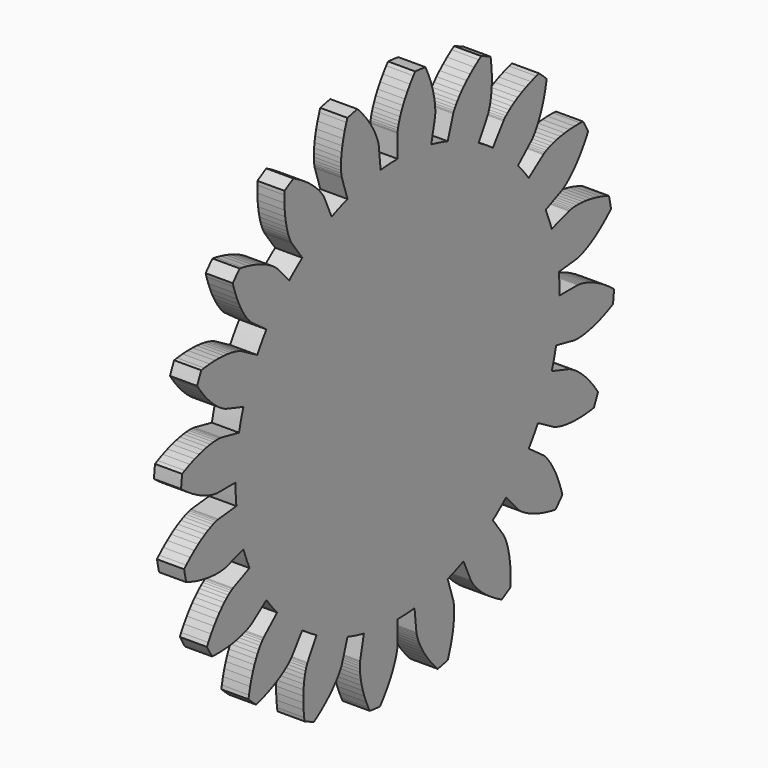
from build123d import *

# Parameters (mm, degrees)
F2_DEPTH = 12.7


# Not quite as in the source:
# - a variable given as a bare number and used for a length is read in inches; the dataset says mm whatever the document's units were


with BuildPart() as f2:
    # F1 (on Right) → F2 (new body)
    with BuildSketch(Plane.YZ):
        with BuildLine():
            ThreePointArc((92.7008893406, -19.704182302), (94.2527120653, -9.9063592233), (94.7718823529, 0))
            ThreePointArc((94.7718823529, 0), (94.6420007819, 4.9599770879), (94.2527120653, 9.9063592233))
            ThreePointArc((94.2527120653, 9.9063592233), (92.7008893406, 19.704182302), (90.1334162733, 29.286122236))
            ThreePointArc((90.1334162733, 29.286122236), (88.477174347, 33.9632051534), (86.5784226358, 38.5471972862))
            ThreePointArc((86.5784226358, 38.5471972862), (82.0748576821, 47.3859411765), (76.6720634124, 55.7055147791))
            ThreePointArc((76.6720634124, 55.7055147791), (73.6515856303, 59.6418780629), (70.4292339713, 63.4147671046))
            ThreePointArc((70.4292339713, 63.4147671046), (63.4147671046, 70.4292339713), (55.7055147791, 76.6720634124))
            ThreePointArc((55.7055147791, 76.6720634124), (51.6164665513, 79.4823883982), (47.3859411765, 82.0748576821))
            ThreePointArc((47.3859411765, 82.0748576821), (38.5471972862, 86.5784226358), (29.286122236, 90.1334162733))
            ThreePointArc((29.286122236, 90.1334162733), (24.5287680932, 91.5426087707), (19.704182302, 92.7008893406))
            ThreePointArc((19.704182302, 92.7008893406), (9.9063592233, 94.2527120653), (0, 94.7718823529))
            ThreePointArc((0, 94.7718823529), (-4.9599770879, 94.6420007819), (-9.9063592233, 94.2527120653))
            ThreePointArc((-9.9063592233, 94.2527120653), (-19.704182302, 92.7008893406), (-29.286122236, 90.1334162733))
            ThreePointArc((-29.286122236, 90.1334162733), (-33.9632051534, 88.477174347), (-38.5471972862, 86.5784226358))
            ThreePointArc((-38.5471972862, 86.5784226358), (-47.3859411765, 82.0748576821), (-55.7055147791, 76.6720634124))
            ThreePointArc((-55.7055147791, 76.6720634124), (-59.6418780629, 73.6515856303), (-63.4147671046, 70.4292339713))
            ThreePointArc((-63.4147671046, 70.4292339713), (-70.4292339713, 63.4147671046), (-76.6720634124, 55.7055147791))
            ThreePointArc((-76.6720634124, 55.7055147791), (-79.4823883982, 51.6164665513), (-82.0748576821, 47.3859411765))
            ThreePointArc((-82.0748576821, 47.3859411765), (-86.5784226358, 38.5471972862), (-90.1334162733, 29.286122236))
            ThreePointArc((-90.1334162733, 29.286122236), (-91.5426087707, 24.5287680932), (-92.7008893406, 19.704182302))
            ThreePointArc((-92.7008893406, 19.704182302), (-94.2527120653, 9.9063592233), (-94.7718823529, 0))
            ThreePointArc((-94.7718823529, 0), (-94.6420007819, -4.9599770879), (-94.2527120653, -9.9063592233))
            ThreePointArc((-94.2527120653, -9.9063592233), (-92.7008893406, -19.704182302), (-90.1334162733, -29.286122236))
            ThreePointArc((-90.1334162733, -29.286122236), (-88.477174347, -33.9632051534), (-86.5784226358, -38.5471972862))
            ThreePointArc((-86.5784226358, -38.5471972862), (-82.0748576821, -47.3859411765), (-76.6720634124, -55.7055147791))
            ThreePointArc((-76.6720634124, -55.7055147791), (-73.6515856303, -59.6418780629), (-70.4292339713, -63.4147671046))
            ThreePointArc((-70.4292339713, -63.4147671046), (-63.4147671046, -70.4292339713), (-55.7055147791, -76.6720634124))
            ThreePointArc((-55.7055147791, -76.6720634124), (-51.6164665513, -79.4823883982), (-47.3859411765, -82.0748576821))
            ThreePointArc((-47.3859411765, -82.0748576821), (-38.5471972862, -86.5784226358), (-29.286122236, -90.1334162733))
            ThreePointArc((-29.286122236, -90.1334162733), (-24.5287680932, -91.5426087707), (-19.704182302, -92.7008893406))
            ThreePointArc((-19.704182302, -92.7008893406), (-9.9063592233, -94.2527120653), (0, -94.7718823529))
            ThreePointArc((0, -94.7718823529), (4.9599770879, -94.6420007819), (9.9063592233, -94.2527120653))
            ThreePointArc((9.9063592233, -94.2527120653), (19.704182302, -92.7008893406), (29.286122236, -90.1334162733))
            ThreePointArc((29.286122236, -90.1334162733), (33.9632051534, -88.477174347), (38.5471972862, -86.5784226358))
            ThreePointArc((38.5471972862, -86.5784226358), (47.3859411765, -82.0748576821), (55.7055147791, -76.6720634124))
            ThreePointArc((55.7055147791, -76.6720634124), (59.6418780629, -73.6515856303), (63.4147671046, -70.4292339713))
            ThreePointArc((63.4147671046, -70.4292339713), (70.4292339713, -63.4147671046), (76.6720634124, -55.7055147791))
            ThreePointArc((76.6720634124, -55.7055147791), (79.4823883982, -51.6164665513), (82.0748576821, -47.3859411765))
            ThreePointArc((82.0748576821, -47.3859411765), (86.5784226358, -38.5471972862), (90.1334162733, -29.286122236))
            ThreePointArc((90.1334162733, -29.286122236), (91.5426087707, -24.5287680932), (92.7008893406, -19.704182302))
        make_face()
        with BuildLine():
            Line((-100.1470591498, -32.5397520376), (-90.1334162733, -29.286122236))
            ThreePointArc((-90.1334162733, -29.286122236), (-92.7008893406, -19.704182302), (-94.2527120653, -9.9063592233))
            Line((-94.2527120653, -9.9063592233), (-104.7240004928, -11.0069359858))
            Line((-104.7240004928, -11.0069359858), (-104.8543651896, -11.0250483896))
            Line((-104.8543651896, -11.0250483896), (-105.2426468777, -11.0967061046))
            Line((-105.2426468777, -11.0967061046), (-105.8831717727, -11.2476177493))
            Line((-105.8831717727, -11.2476177493), (-106.7683476445, -11.5030264298))
            Line((-106.7683476445, -11.5030264298), (-107.8886977686, -11.8875826074))
            Line((-107.8886977686, -11.8875826074), (-109.2329027705, -12.4252192764))
            Line((-109.2329027705, -12.4252192764), (-110.7878502107, -13.1390299218))
            Line((-110.7878502107, -13.1390299218), (-112.5386917362, -14.051149717))
            Line((-112.5386917362, -14.051149717), (-114.4689075917, -15.1826404116))
            Line((-114.4689075917, -15.1826404116), (-116.5603782638, -16.5533793458))
            Line((-116.5603782638, -16.5533793458), (-118.793463, -18.1819530161))
            Line((-118.793463, -18.1819530161), (-121.1470849264, -20.0855555985))
            Line((-121.1470849264, -20.0855555985), (-123.5988224587, -22.2798928209))
            Line((-123.5988224587, -22.2798928209), (-124.8108146855, -23.4789381691))
            ThreePointArc((-124.8108146855, -23.4789381691), (-124.2247452932, -26.4047847339), (-123.5700973145, -29.3160544701))
            Line((-123.5700973145, -29.3160544701), (-121.9751916412, -29.9184752517))
            Line((-121.9751916412, -29.9184752517), (-118.8429005996, -30.9258905601))
            Line((-118.8429005996, -30.9258905601), (-115.9184950556, -31.707613771))
            Line((-115.9184950556, -31.707613771), (-113.2160700507, -32.2871124607))
            Line((-113.2160700507, -32.2871124607), (-110.7478867658, -32.6886670274))
            Line((-110.7478867658, -32.6886670274), (-108.5243281119, -32.9372456942))
            Line((-108.5243281119, -32.9372456942), (-106.5538622456, -33.0583771854))
            Line((-106.5538622456, -33.0583771854), (-104.843014129, -33.0780215561))
            Line((-104.843014129, -33.0780215561), (-103.3963452215, -33.0224396629))
            Line((-103.3963452215, -33.0224396629), (-102.2164413659, -32.9180617635))
            Line((-102.2164413659, -32.9180617635), (-101.3039088997, -32.7913557409))
            Line((-101.3039088997, -32.7913557409), (-100.6573789956, -32.6686954428))
            Line((-100.6573789956, -32.6686954428), (-100.2735202047, -32.5762296325))
            Line((-100.2735202047, -32.5762296325), (-100.1470591498, -32.5397520376))
        make_face()
        with BuildLine():
            Line((-85.1901768198, -61.8942864279), (-76.6720634124, -55.7055147791))
            ThreePointArc((-76.6720634124, -55.7055147791), (-82.0748576821, -47.3859411765), (-86.5784226358, -38.5471972862))
            Line((-86.5784226358, -38.5471972862), (-96.1971128056, -42.8297140649))
            Line((-96.1971128056, -42.8297140649), (-96.3154999594, -42.8872248914))
            Line((-96.3154999594, -42.8872248914), (-96.6626343373, -43.0753610684))
            Line((-96.6626343373, -43.0753610684), (-97.2251754497, -43.4168196494))
            Line((-97.2251754497, -43.4168196494), (-97.9881021078, -43.9332621267))
            Line((-97.9881021078, -43.9332621267), (-98.9347839997, -44.6452040132))
            Line((-98.9347839997, -44.6452040132), (-100.0470600584, -45.5719090602))
            Line((-100.0470600584, -45.5719090602), (-101.3053233338, -46.7312885103))
            Line((-101.3053233338, -46.7312885103), (-102.6886120579, -48.139805771))
            Line((-102.6886120579, -48.139805771), (-104.1747065717, -49.8123868714))
            Line((-104.1747065717, -49.8123868714), (-105.7402317574, -51.7623370478))
            Line((-105.7402317574, -51.7623370478), (-107.3607646065, -54.0012637826))
            Line((-107.3607646065, -54.0012637826), (-109.010946528, -56.5390065966))
            Line((-109.010946528, -56.5390065966), (-110.6645999913, -59.3835738742))
            Line((-110.6645999913, -59.3835738742), (-111.4467477066, -60.898459961))
            ThreePointArc((-111.4467477066, -60.898459961), (-109.9852262806, -63.5), (-108.4629872309, -66.0664847026))
            Line((-108.4629872309, -66.0664847026), (-106.7599835382, -66.146567955))
            Line((-106.7599835382, -66.146567955), (-103.4696892814, -66.1367456855))
            Line((-103.4696892814, -66.1367456855), (-100.4468485755, -65.9765176277))
            Line((-100.4468485755, -65.9765176277), (-97.6976147214, -65.6925583801))
            Line((-97.6976147214, -65.6925583801), (-95.2261457396, -65.3117488872))
            Line((-95.2261457396, -65.3117488872), (-93.0346007599, -64.861043836))
            Line((-93.0346007599, -64.861043836), (-91.1231446684, -64.3673392905))
            Line((-91.1231446684, -64.3673392905), (-89.4899609743, -63.8573410545))
            Line((-89.4899609743, -63.8573410545), (-88.1312728324, -63.3574342551))
            Line((-88.1312728324, -63.3574342551), (-87.0413721267, -62.8935546306))
            Line((-87.0413721267, -62.8935546306), (-86.2126564928, -62.4910620021))
            Line((-86.2126564928, -62.4910620021), (-85.6356741311, -62.1746163987))
            Line((-85.6356741311, -62.1746163987), (-85.2991762334, -61.9680572974))
            Line((-85.2991762334, -61.9680572974), (-85.1901768198, -61.8942864279))
        make_face()
        with BuildLine():
            Line((-61.8942864279, -85.1901768198), (-55.7055147791, -76.6720634124))
            ThreePointArc((-55.7055147791, -76.6720634124), (-63.4147671046, -70.4292339713), (-70.4292339713, -63.4147671046))
            Line((-70.4292339713, -63.4147671046), (-78.2537814723, -70.4600213192))
            Line((-78.2537814723, -70.4600213192), (-78.3486025236, -70.5513010079))
            Line((-78.3486025236, -70.5513010079), (-78.6206096598, -70.8374995671))
            Line((-78.6206096598, -70.8374995671), (-79.050101546, -71.3360807394))
            Line((-79.050101546, -71.3360807394), (-79.6160984135, -72.0630040255))
            Line((-79.6160984135, -72.0630040255), (-80.2964442538, -73.0326417888))
            Line((-80.2964442538, -73.0326417888), (-81.0679140391, -74.257702867))
            Line((-81.0679140391, -74.257702867), (-81.9063255732, -75.7491629834))
            Line((-81.9063255732, -75.7491629834), (-82.7866555578, -77.5162022264))
            Line((-82.7866555578, -77.5162022264), (-83.6831594445, -79.5661498409))
            Line((-83.6831594445, -79.5661498409), (-84.5694946311, -81.9044365502))
            Line((-84.5694946311, -81.9044365502), (-85.4188465469, -84.5345546011))
            Line((-85.4188465469, -84.5345546011), (-86.2040571595, -87.4580256986))
            Line((-86.2040571595, -87.4580256986), (-86.8977554311, -90.6743769669))
            Line((-86.8977554311, -90.6743769669), (-87.1734965671, -92.3568161874))
            ThreePointArc((-87.1734965671, -92.3568161874), (-84.9795870076, -94.3793928356), (-82.738764251, -96.3498671001))
            Line((-82.738764251, -96.3498671001), (-81.0943644059, -95.8997737166))
            Line((-81.0943644059, -95.8997737166), (-77.9681438606, -94.8736753414))
            Line((-77.9681438606, -94.8736753414), (-75.1427647024, -93.7871802535))
            Line((-75.1427647024, -93.7871802535), (-72.6158361638, -92.6675589783))
            Line((-72.6158361638, -92.6675589783), (-70.3830060888, -91.5416617121))
            Line((-70.3830060888, -91.5416617121), (-68.4379984754, -90.4357910937))
            Line((-68.4379984754, -90.4357910937), (-66.7726587987, -89.3755777522))
            Line((-66.7726587987, -89.3755777522), (-65.3770069262, -88.3858590901))
            Line((-65.3770069262, -88.3858590901), (-64.2392974119, -87.4905617451))
            Line((-64.2392974119, -87.4905617451), (-63.3460869309, -86.7125881653))
            Line((-63.3460869309, -86.7125881653), (-62.6823085893, -86.0737077138))
            Line((-62.6823085893, -86.0737077138), (-62.2313528238, -85.5944527054))
            Line((-62.2313528238, -85.5944527054), (-61.9751545781, -85.2940197571))
            Line((-61.9751545781, -85.2940197571), (-61.8942864279, -85.1901768198))
        make_face()
        with BuildLine():
            Line((-32.5397520376, -100.1470591498), (-29.286122236, -90.1334162733))
            ThreePointArc((-29.286122236, -90.1334162733), (-38.5471972862, -86.5784226358), (-47.3859411765, -82.0748576821))
            Line((-47.3859411765, -82.0748576821), (-52.6504247823, -91.193210763))
            Line((-52.6504247823, -91.193210763), (-52.712397986, -91.309324222))
            Line((-52.712397986, -91.309324222), (-52.8826519268, -91.6655700544))
            Line((-52.8826519268, -91.6655700544), (-53.1370529285, -92.272469219))
            Line((-53.1370529285, -92.272469219), (-53.4507162886, -93.1387169979))
            Line((-53.4507162886, -93.1387169979), (-53.798129086, -94.2711357378))
            Line((-53.798129086, -94.2711357378), (-54.1532757602, -95.6746353334))
            Line((-54.1532757602, -95.6746353334), (-54.4897659907, -97.3521816082))
            Line((-54.4897659907, -97.3521816082), (-54.7809644032, -99.3047727207))
            Line((-54.7809644032, -99.3047727207), (-55.000121616, -101.531423694))
            Line((-55.000121616, -101.531423694), (-55.12050614, -104.0291591412))
            Line((-55.12050614, -104.0291591412), (-55.1155366392, -106.7930142284))
            Line((-55.1155366392, -106.7930142284), (-54.9589140573, -109.8160438893))
            Line((-54.9589140573, -109.8160438893), (-54.624753117, -113.0893402766))
            Line((-54.624753117, -113.0893402766), (-54.3670962101, -114.7746437576))
            ThreePointArc((-54.3670962101, -114.7746437576), (-51.6555536706, -116.0202731206), (-48.9154945515, -117.2018531969))
            Line((-48.9154945515, -117.2018531969), (-47.4906638679, -116.2656414539))
            Line((-47.4906638679, -116.2656414539), (-44.8345332828, -114.3237086311))
            Line((-44.8345332828, -114.3237086311), (-42.4831834698, -112.4173002224))
            Line((-42.4831834698, -112.4173002224), (-40.4259136183, -110.5716132508))
            Line((-40.4259136183, -110.5716132508), (-38.6502874148, -108.8108388804))
            Line((-38.6502874148, -108.8108388804), (-37.1422080646, -107.1580530158))
            Line((-37.1422080646, -107.1580530158), (-35.8859998534, -105.6351119473))
            Line((-35.8859998534, -105.6351119473), (-34.8644959317, -104.2625534176))
            Line((-34.8644959317, -104.2625534176), (-34.0591319791, -103.059503469))
            Line((-34.0591319791, -103.059503469), (-33.4500453881, -102.0435894082))
            Line((-33.4500453881, -102.0435894082), (-33.0161795879, -101.2308592037))
            Line((-33.0161795879, -101.2308592037), (-32.7353931107, -100.6357076096))
            Line((-32.7353931107, -100.6357076096), (-32.5845729864, -100.2708092847))
            Line((-32.5845729864, -100.2708092847), (-32.5397520376, -100.1470591498))
        make_face()
        with BuildLine():
            Line((0, -105.3008495645), (0, -94.7718823529))
            ThreePointArc((0, -94.7718823529), (-9.9063592233, -94.2527120653), (-19.704182302, -92.7008893406))
            Line((-19.704182302, -92.7008893406), (-21.8932776775, -102.9997733568))
            Line((-21.8932776775, -102.9997733568), (-21.9163366646, -103.1293545918))
            Line((-21.9163366646, -103.1293545918), (-21.9681717681, -103.5207758731))
            Line((-21.9681717681, -103.5207758731), (-22.0225793428, -104.1765855112))
            Line((-22.0225793428, -104.1765855112), (-22.0532056403, -105.0973634149))
            Line((-22.0532056403, -105.0973634149), (-22.0336782097, -106.2817140951))
            Line((-22.0336782097, -106.2817140951), (-21.9377375418, -107.7262678889))
            Line((-21.9377375418, -107.7262678889), (-21.7393684604, -109.4256904046))
            Line((-21.7393684604, -109.4256904046), (-21.4129307714, -111.3727001641))
            Line((-21.4129307714, -111.3727001641), (-20.9332886754, -113.558094385))
            Line((-20.9332886754, -113.558094385), (-20.2759384608, -115.9707828218))
            Line((-20.2759384608, -115.9707828218), (-19.4171339927, -118.5978295523))
            Line((-19.4171339927, -118.5978295523), (-18.3340095258, -121.4245025708))
            Line((-18.3340095258, -121.4245025708), (-17.0046993748, -124.4343310203))
            Line((-17.0046993748, -124.4343310203), (-16.2388656782, -125.9575295149))
            ThreePointArc((-16.2388656782, -125.9575295149), (-13.275114835, -126.3042807118), (-10.3040354309, -126.5813053094))
            Line((-10.3040354309, -126.5813053094), (-9.2382462636, -125.2506181353))
            Line((-9.2382462636, -125.2506181353), (-7.3122062067, -122.5829407799))
            Line((-7.3122062067, -122.5829407799), (-5.6650522415, -120.0432315881))
            Line((-5.6650522415, -120.0432315881), (-4.2788209839, -117.6521476207))
            Line((-4.2788209839, -117.6521476207), (-3.1342093163, -115.4288530094))
            Line((-3.1342093163, -115.4288530094), (-2.2106795434, -113.3909380948))
            Line((-2.2106795434, -113.3909380948), (-1.4865692099, -111.5543453819))
            Line((-1.4865692099, -111.5543453819), (-0.9392051602, -109.9333025766))
            Line((-0.9392051602, -109.9333025766), (-0.5450214043, -108.5402629356))
            Line((-0.5450214043, -108.5402629356), (-0.2796803426, -107.3858531403))
            Line((-0.2796803426, -107.3858531403), (-0.1181968911, -106.4788288778))
            Line((-0.1181968911, -106.4788288778), (-0.0350650391, -105.8260382829))
            Line((-0.0350650391, -105.8260382829), (-0.0043863607, -105.4323933716))
            Line((-0.0043863607, -105.4323933716), (0, -105.3008495645))
        make_face()
        with BuildLine():
            Line((32.5397520376, -100.1470591498), (29.286122236, -90.1334162733))
            ThreePointArc((29.286122236, -90.1334162733), (19.704182302, -92.7008893406), (9.9063592233, -94.2527120653))
            Line((9.9063592233, -94.2527120653), (11.0069359858, -104.7240004928))
            Line((11.0069359858, -104.7240004928), (11.0250483896, -104.8543651896))
            Line((11.0250483896, -104.8543651896), (11.0967061046, -105.2426468777))
            Line((11.0967061046, -105.2426468777), (11.2476177493, -105.8831717727))
            Line((11.2476177493, -105.8831717727), (11.5030264298, -106.7683476445))
            Line((11.5030264298, -106.7683476445), (11.8875826074, -107.8886977686))
            Line((11.8875826074, -107.8886977686), (12.4252192764, -109.2329027705))
            Line((12.4252192764, -109.2329027705), (13.1390299218, -110.7878502107))
            Line((13.1390299218, -110.7878502107), (14.051149717, -112.5386917362))
            Line((14.051149717, -112.5386917362), (15.1826404116, -114.4689075917))
            Line((15.1826404116, -114.4689075917), (16.5533793458, -116.5603782638))
            Line((16.5533793458, -116.5603782638), (18.1819530161, -118.793463))
            Line((18.1819530161, -118.793463), (20.0855555985, -121.1470849264))
            Line((20.0855555985, -121.1470849264), (22.2798928209, -123.5988224587))
            Line((22.2798928209, -123.5988224587), (23.4789381691, -124.8108146855))
            ThreePointArc((23.4789381691, -124.8108146855), (26.4047847339, -124.2247452932), (29.3160544701, -123.5700973145))
            Line((29.3160544701, -123.5700973145), (29.9184752517, -121.9751916412))
            Line((29.9184752517, -121.9751916412), (30.9258905601, -118.8429005996))
            Line((30.9258905601, -118.8429005996), (31.707613771, -115.9184950556))
            Line((31.707613771, -115.9184950556), (32.2871124607, -113.2160700507))
            Line((32.2871124607, -113.2160700507), (32.6886670274, -110.7478867658))
            Line((32.6886670274, -110.7478867658), (32.9372456942, -108.5243281119))
            Line((32.9372456942, -108.5243281119), (33.0583771854, -106.5538622456))
            Line((33.0583771854, -106.5538622456), (33.0780215561, -104.843014129))
            Line((33.0780215561, -104.843014129), (33.0224396629, -103.3963452215))
            Line((33.0224396629, -103.3963452215), (32.9180617635, -102.2164413659))
            Line((32.9180617635, -102.2164413659), (32.7913557409, -101.3039088997))
            Line((32.7913557409, -101.3039088997), (32.6686954428, -100.6573789956))
            Line((32.6686954428, -100.6573789956), (32.5762296325, -100.2735202047))
            Line((32.5762296325, -100.2735202047), (32.5397520376, -100.1470591498))
        make_face()
        with BuildLine():
            Line((61.8942864279, -85.1901768198), (55.7055147791, -76.6720634124))
            ThreePointArc((55.7055147791, -76.6720634124), (47.3859411765, -82.0748576821), (38.5471972862, -86.5784226358))
            Line((38.5471972862, -86.5784226358), (42.8297140649, -96.1971128056))
            Line((42.8297140649, -96.1971128056), (42.8872248914, -96.3154999594))
            Line((42.8872248914, -96.3154999594), (43.0753610684, -96.6626343373))
            Line((43.0753610684, -96.6626343373), (43.4168196494, -97.2251754497))
            Line((43.4168196494, -97.2251754497), (43.9332621267, -97.9881021078))
            Line((43.9332621267, -97.9881021078), (44.6452040132, -98.9347839997))
            Line((44.6452040132, -98.9347839997), (45.5719090602, -100.0470600584))
            Line((45.5719090602, -100.0470600584), (46.7312885103, -101.3053233338))
            Line((46.7312885103, -101.3053233338), (48.139805771, -102.6886120579))
            Line((48.139805771, -102.6886120579), (49.8123868714, -104.1747065717))
            Line((49.8123868714, -104.1747065717), (51.7623370478, -105.7402317574))
            Line((51.7623370478, -105.7402317574), (54.0012637826, -107.3607646065))
            Line((54.0012637826, -107.3607646065), (56.5390065966, -109.010946528))
            Line((56.5390065966, -109.010946528), (59.3835738742, -110.6645999913))
            Line((59.3835738742, -110.6645999913), (60.898459961, -111.4467477066))
            ThreePointArc((60.898459961, -111.4467477066), (63.5, -109.9852262806), (66.0664847026, -108.4629872309))
            Line((66.0664847026, -108.4629872309), (66.146567955, -106.7599835382))
            Line((66.146567955, -106.7599835382), (66.1367456855, -103.4696892814))
            Line((66.1367456855, -103.4696892814), (65.9765176277, -100.4468485755))
            Line((65.9765176277, -100.4468485755), (65.6925583801, -97.6976147214))
            Line((65.6925583801, -97.6976147214), (65.3117488872, -95.2261457396))
            Line((65.3117488872, -95.2261457396), (64.861043836, -93.0346007599))
            Line((64.861043836, -93.0346007599), (64.3673392905, -91.1231446684))
            Line((64.3673392905, -91.1231446684), (63.8573410545, -89.4899609743))
            Line((63.8573410545, -89.4899609743), (63.3574342551, -88.1312728324))
            Line((63.3574342551, -88.1312728324), (62.8935546306, -87.0413721267))
            Line((62.8935546306, -87.0413721267), (62.4910620021, -86.2126564928))
            Line((62.4910620021, -86.2126564928), (62.1746163987, -85.6356741311))
            Line((62.1746163987, -85.6356741311), (61.9680572974, -85.2991762334))
            Line((61.9680572974, -85.2991762334), (61.8942864279, -85.1901768198))
        make_face()
        with BuildLine():
            Line((85.1901768198, -61.8942864279), (76.6720634124, -55.7055147791))
            ThreePointArc((76.6720634124, -55.7055147791), (70.4292339713, -63.4147671046), (63.4147671046, -70.4292339713))
            Line((63.4147671046, -70.4292339713), (70.4600213192, -78.2537814723))
            Line((70.4600213192, -78.2537814723), (70.5513010079, -78.3486025236))
            Line((70.5513010079, -78.3486025236), (70.8374995671, -78.6206096598))
            Line((70.8374995671, -78.6206096598), (71.3360807394, -79.050101546))
            Line((71.3360807394, -79.050101546), (72.0630040255, -79.6160984135))
            Line((72.0630040255, -79.6160984135), (73.0326417888, -80.2964442538))
            Line((73.0326417888, -80.2964442538), (74.257702867, -81.0679140391))
            Line((74.257702867, -81.0679140391), (75.7491629834, -81.9063255732))
            Line((75.7491629834, -81.9063255732), (77.5162022264, -82.7866555578))
            Line((77.5162022264, -82.7866555578), (79.5661498409, -83.6831594445))
            Line((79.5661498409, -83.6831594445), (81.9044365502, -84.5694946311))
            Line((81.9044365502, -84.5694946311), (84.5345546011, -85.4188465469))
            Line((84.5345546011, -85.4188465469), (87.4580256986, -86.2040571595))
            Line((87.4580256986, -86.2040571595), (90.6743769669, -86.8977554311))
            Line((90.6743769669, -86.8977554311), (92.3568161874, -87.1734965671))
            ThreePointArc((92.3568161874, -87.1734965671), (94.3793928356, -84.9795870076), (96.3498671001, -82.738764251))
            Line((96.3498671001, -82.738764251), (95.8997737166, -81.0943644059))
            Line((95.8997737166, -81.0943644059), (94.8736753414, -77.9681438606))
            Line((94.8736753414, -77.9681438606), (93.7871802535, -75.1427647024))
            Line((93.7871802535, -75.1427647024), (92.6675589783, -72.6158361638))
            Line((92.6675589783, -72.6158361638), (91.5416617121, -70.3830060888))
            Line((91.5416617121, -70.3830060888), (90.4357910937, -68.4379984754))
            Line((90.4357910937, -68.4379984754), (89.3755777522, -66.7726587987))
            Line((89.3755777522, -66.7726587987), (88.3858590901, -65.3770069262))
            Line((88.3858590901, -65.3770069262), (87.4905617451, -64.2392974119))
            Line((87.4905617451, -64.2392974119), (86.7125881653, -63.3460869309))
            Line((86.7125881653, -63.3460869309), (86.0737077138, -62.6823085893))
            Line((86.0737077138, -62.6823085893), (85.5944527054, -62.2313528238))
            Line((85.5944527054, -62.2313528238), (85.2940197571, -61.9751545781))
            Line((85.2940197571, -61.9751545781), (85.1901768198, -61.8942864279))
        make_face()
        with BuildLine():
            Line((100.1470591498, -32.5397520376), (90.1334162733, -29.286122236))
            ThreePointArc((90.1334162733, -29.286122236), (86.5784226358, -38.5471972862), (82.0748576821, -47.3859411765))
            Line((82.0748576821, -47.3859411765), (91.193210763, -52.6504247823))
            Line((91.193210763, -52.6504247823), (91.309324222, -52.712397986))
            Line((91.309324222, -52.712397986), (91.6655700544, -52.8826519268))
            Line((91.6655700544, -52.8826519268), (92.272469219, -53.1370529285))
            Line((92.272469219, -53.1370529285), (93.1387169979, -53.4507162886))
            Line((93.1387169979, -53.4507162886), (94.2711357378, -53.798129086))
            Line((94.2711357378, -53.798129086), (95.6746353334, -54.1532757602))
            Line((95.6746353334, -54.1532757602), (97.3521816082, -54.4897659907))
            Line((97.3521816082, -54.4897659907), (99.3047727207, -54.7809644032))
            Line((99.3047727207, -54.7809644032), (101.531423694, -55.000121616))
            Line((101.531423694, -55.000121616), (104.0291591412, -55.12050614))
            Line((104.0291591412, -55.12050614), (106.7930142284, -55.1155366392))
            Line((106.7930142284, -55.1155366392), (109.8160438893, -54.9589140573))
            Line((109.8160438893, -54.9589140573), (113.0893402766, -54.624753117))
            Line((113.0893402766, -54.624753117), (114.7746437576, -54.3670962101))
            ThreePointArc((114.7746437576, -54.3670962101), (116.0202731206, -51.6555536706), (117.2018531969, -48.9154945515))
            Line((117.2018531969, -48.9154945515), (116.2656414539, -47.4906638679))
            Line((116.2656414539, -47.4906638679), (114.3237086311, -44.8345332828))
            Line((114.3237086311, -44.8345332828), (112.4173002224, -42.4831834698))
            Line((112.4173002224, -42.4831834698), (110.5716132508, -40.4259136183))
            Line((110.5716132508, -40.4259136183), (108.8108388804, -38.6502874148))
            Line((108.8108388804, -38.6502874148), (107.1580530158, -37.1422080646))
            Line((107.1580530158, -37.1422080646), (105.6351119473, -35.8859998534))
            Line((105.6351119473, -35.8859998534), (104.2625534176, -34.8644959317))
            Line((104.2625534176, -34.8644959317), (103.059503469, -34.0591319791))
            Line((103.059503469, -34.0591319791), (102.0435894082, -33.4500453881))
            Line((102.0435894082, -33.4500453881), (101.2308592037, -33.0161795879))
            Line((101.2308592037, -33.0161795879), (100.6357076096, -32.7353931107))
            Line((100.6357076096, -32.7353931107), (100.2708092847, -32.5845729864))
            Line((100.2708092847, -32.5845729864), (100.1470591498, -32.5397520376))
        make_face()
        with BuildLine():
            Line((105.3008495645, 0), (94.7718823529, 0))
            ThreePointArc((94.7718823529, 0), (94.2527120653, -9.9063592233), (92.7008893406, -19.704182302))
            Line((92.7008893406, -19.704182302), (102.9997733568, -21.8932776775))
            Line((102.9997733568, -21.8932776775), (103.1293545918, -21.9163366646))
            Line((103.1293545918, -21.9163366646), (103.5207758731, -21.9681717681))
            Line((103.5207758731, -21.9681717681), (104.1765855112, -22.0225793428))
            Line((104.1765855112, -22.0225793428), (105.0973634149, -22.0532056403))
            Line((105.0973634149, -22.0532056403), (106.2817140951, -22.0336782097))
            Line((106.2817140951, -22.0336782097), (107.7262678889, -21.9377375418))
            Line((107.7262678889, -21.9377375418), (109.4256904046, -21.7393684604))
            Line((109.4256904046, -21.7393684604), (111.3727001641, -21.4129307714))
            Line((111.3727001641, -21.4129307714), (113.558094385, -20.9332886754))
            Line((113.558094385, -20.9332886754), (115.9707828218, -20.2759384608))
            Line((115.9707828218, -20.2759384608), (118.5978295523, -19.4171339927))
            Line((118.5978295523, -19.4171339927), (121.4245025708, -18.3340095258))
            Line((121.4245025708, -18.3340095258), (124.4343310203, -17.0046993748))
            Line((124.4343310203, -17.0046993748), (125.9575295149, -16.2388656782))
            ThreePointArc((125.9575295149, -16.2388656782), (126.3042807118, -13.275114835), (126.5813053094, -10.3040354309))
            Line((126.5813053094, -10.3040354309), (125.2506181353, -9.2382462636))
            Line((125.2506181353, -9.2382462636), (122.5829407799, -7.3122062067))
            Line((122.5829407799, -7.3122062067), (120.0432315881, -5.6650522415))
            Line((120.0432315881, -5.6650522415), (117.6521476207, -4.2788209839))
            Line((117.6521476207, -4.2788209839), (115.4288530094, -3.1342093163))
            Line((115.4288530094, -3.1342093163), (113.3909380948, -2.2106795434))
            Line((113.3909380948, -2.2106795434), (111.5543453819, -1.4865692099))
            Line((111.5543453819, -1.4865692099), (109.9333025766, -0.9392051602))
            Line((109.9333025766, -0.9392051602), (108.5402629356, -0.5450214043))
            Line((108.5402629356, -0.5450214043), (107.3858531403, -0.2796803426))
            Line((107.3858531403, -0.2796803426), (106.4788288778, -0.1181968911))
            Line((106.4788288778, -0.1181968911), (105.8260382829, -0.0350650391))
            Line((105.8260382829, -0.0350650391), (105.4323933716, -0.0043863607))
            Line((105.4323933716, -0.0043863607), (105.3008495645, 0))
        make_face()
        with BuildLine():
            ThreePointArc((90.1334162733, 29.286122236), (92.7008893406, 19.704182302), (94.2527120653, 9.9063592233))
            Line((94.2527120653, 9.9063592233), (104.7240004928, 11.0069359858))
            Line((104.7240004928, 11.0069359858), (104.8543651896, 11.0250483896))
            Line((104.8543651896, 11.0250483896), (105.2426468777, 11.0967061046))
            Line((105.2426468777, 11.0967061046), (105.8831717727, 11.2476177493))
            Line((105.8831717727, 11.2476177493), (106.7683476445, 11.5030264298))
            Line((106.7683476445, 11.5030264298), (107.8886977686, 11.8875826074))
            Line((107.8886977686, 11.8875826074), (109.2329027705, 12.4252192764))
            Line((109.2329027705, 12.4252192764), (110.7878502107, 13.1390299218))
            Line((110.7878502107, 13.1390299218), (112.5386917362, 14.051149717))
            Line((112.5386917362, 14.051149717), (114.4689075917, 15.1826404116))
            Line((114.4689075917, 15.1826404116), (116.5603782638, 16.5533793458))
            Line((116.5603782638, 16.5533793458), (118.793463, 18.1819530161))
            Line((118.793463, 18.1819530161), (121.1470849264, 20.0855555985))
            Line((121.1470849264, 20.0855555985), (123.5988224587, 22.2798928209))
            Line((123.5988224587, 22.2798928209), (124.8108146855, 23.4789381691))
            ThreePointArc((124.8108146855, 23.4789381691), (124.2247452932, 26.4047847339), (123.5700973145, 29.3160544701))
            Line((123.5700973145, 29.3160544701), (121.9751916412, 29.9184752517))
            Line((121.9751916412, 29.9184752517), (118.8429005996, 30.9258905601))
            Line((118.8429005996, 30.9258905601), (115.9184950556, 31.707613771))
            Line((115.9184950556, 31.707613771), (113.2160700507, 32.2871124607))
            Line((113.2160700507, 32.2871124607), (110.7478867658, 32.6886670274))
            Line((110.7478867658, 32.6886670274), (108.5243281119, 32.9372456942))
            Line((108.5243281119, 32.9372456942), (106.5538622456, 33.0583771854))
            Line((106.5538622456, 33.0583771854), (104.843014129, 33.0780215561))
            Line((104.843014129, 33.0780215561), (103.3963452215, 33.0224396629))
            Line((103.3963452215, 33.0224396629), (102.2164413659, 32.9180617635))
            Line((102.2164413659, 32.9180617635), (101.3039088997, 32.7913557409))
            Line((101.3039088997, 32.7913557409), (100.6573789956, 32.6686954428))
            Line((100.6573789956, 32.6686954428), (100.2735202047, 32.5762296325))
            Line((100.2735202047, 32.5762296325), (100.1470591498, 32.5397520376))
            Line((100.1470591498, 32.5397520376), (90.1334162733, 29.286122236))
        make_face()
        with BuildLine():
            ThreePointArc((76.6720634124, 55.7055147791), (82.0748576821, 47.3859411765), (86.5784226358, 38.5471972862))
            Line((86.5784226358, 38.5471972862), (96.1971128056, 42.8297140649))
            Line((96.1971128056, 42.8297140649), (96.3154999594, 42.8872248914))
            Line((96.3154999594, 42.8872248914), (96.6626343373, 43.0753610684))
            Line((96.6626343373, 43.0753610684), (97.2251754497, 43.4168196494))
            Line((97.2251754497, 43.4168196494), (97.9881021078, 43.9332621267))
            Line((97.9881021078, 43.9332621267), (98.9347839997, 44.6452040132))
            Line((98.9347839997, 44.6452040132), (100.0470600584, 45.5719090602))
            Line((100.0470600584, 45.5719090602), (101.3053233338, 46.7312885103))
            Line((101.3053233338, 46.7312885103), (102.6886120579, 48.139805771))
            Line((102.6886120579, 48.139805771), (104.1747065717, 49.8123868714))
            Line((104.1747065717, 49.8123868714), (105.7402317574, 51.7623370478))
            Line((105.7402317574, 51.7623370478), (107.3607646065, 54.0012637826))
            Line((107.3607646065, 54.0012637826), (109.010946528, 56.5390065966))
            Line((109.010946528, 56.5390065966), (110.6645999913, 59.3835738742))
            Line((110.6645999913, 59.3835738742), (111.4467477066, 60.898459961))
            ThreePointArc((111.4467477066, 60.898459961), (109.9852262806, 63.5), (108.4629872309, 66.0664847026))
            Line((108.4629872309, 66.0664847026), (106.7599835382, 66.146567955))
            Line((106.7599835382, 66.146567955), (103.4696892814, 66.1367456855))
            Line((103.4696892814, 66.1367456855), (100.4468485755, 65.9765176277))
            Line((100.4468485755, 65.9765176277), (97.6976147214, 65.6925583801))
            Line((97.6976147214, 65.6925583801), (95.2261457396, 65.3117488872))
            Line((95.2261457396, 65.3117488872), (93.0346007599, 64.861043836))
            Line((93.0346007599, 64.861043836), (91.1231446684, 64.3673392905))
            Line((91.1231446684, 64.3673392905), (89.4899609743, 63.8573410545))
            Line((89.4899609743, 63.8573410545), (88.1312728324, 63.3574342551))
            Line((88.1312728324, 63.3574342551), (87.0413721267, 62.8935546306))
            Line((87.0413721267, 62.8935546306), (86.2126564928, 62.4910620021))
            Line((86.2126564928, 62.4910620021), (85.6356741311, 62.1746163987))
            Line((85.6356741311, 62.1746163987), (85.2991762334, 61.9680572974))
            Line((85.2991762334, 61.9680572974), (85.1901768198, 61.8942864279))
            Line((85.1901768198, 61.8942864279), (76.6720634124, 55.7055147791))
        make_face()
        with BuildLine():
            ThreePointArc((55.7055147791, 76.6720634124), (63.4147671046, 70.4292339713), (70.4292339713, 63.4147671046))
            Line((70.4292339713, 63.4147671046), (78.2537814723, 70.4600213192))
            Line((78.2537814723, 70.4600213192), (78.3486025236, 70.5513010079))
            Line((78.3486025236, 70.5513010079), (78.6206096598, 70.8374995671))
            Line((78.6206096598, 70.8374995671), (79.050101546, 71.3360807394))
            Line((79.050101546, 71.3360807394), (79.6160984135, 72.0630040255))
            Line((79.6160984135, 72.0630040255), (80.2964442538, 73.0326417888))
            Line((80.2964442538, 73.0326417888), (81.0679140391, 74.257702867))
            Line((81.0679140391, 74.257702867), (81.9063255732, 75.7491629834))
            Line((81.9063255732, 75.7491629834), (82.7866555578, 77.5162022264))
            Line((82.7866555578, 77.5162022264), (83.6831594445, 79.5661498409))
            Line((83.6831594445, 79.5661498409), (84.5694946311, 81.9044365502))
            Line((84.5694946311, 81.9044365502), (85.4188465469, 84.5345546011))
            Line((85.4188465469, 84.5345546011), (86.2040571595, 87.4580256986))
            Line((86.2040571595, 87.4580256986), (86.8977554311, 90.6743769669))
            Line((86.8977554311, 90.6743769669), (87.1734965671, 92.3568161874))
            ThreePointArc((87.1734965671, 92.3568161874), (84.9795870076, 94.3793928356), (82.738764251, 96.3498671001))
            Line((82.738764251, 96.3498671001), (81.0943644059, 95.8997737166))
            Line((81.0943644059, 95.8997737166), (77.9681438606, 94.8736753414))
            Line((77.9681438606, 94.8736753414), (75.1427647024, 93.7871802535))
            Line((75.1427647024, 93.7871802535), (72.6158361638, 92.6675589783))
            Line((72.6158361638, 92.6675589783), (70.3830060888, 91.5416617121))
            Line((70.3830060888, 91.5416617121), (68.4379984754, 90.4357910937))
            Line((68.4379984754, 90.4357910937), (66.7726587987, 89.3755777522))
            Line((66.7726587987, 89.3755777522), (65.3770069262, 88.3858590901))
            Line((65.3770069262, 88.3858590901), (64.2392974119, 87.4905617451))
            Line((64.2392974119, 87.4905617451), (63.3460869309, 86.7125881653))
            Line((63.3460869309, 86.7125881653), (62.6823085893, 86.0737077138))
            Line((62.6823085893, 86.0737077138), (62.2313528238, 85.5944527054))
            Line((62.2313528238, 85.5944527054), (61.9751545781, 85.2940197571))
            Line((61.9751545781, 85.2940197571), (61.8942864279, 85.1901768198))
            Line((61.8942864279, 85.1901768198), (55.7055147791, 76.6720634124))
        make_face()
        with BuildLine():
            ThreePointArc((29.286122236, 90.1334162733), (38.5471972862, 86.5784226358), (47.3859411765, 82.0748576821))
            Line((47.3859411765, 82.0748576821), (52.6504247823, 91.193210763))
            Line((52.6504247823, 91.193210763), (52.712397986, 91.309324222))
            Line((52.712397986, 91.309324222), (52.8826519268, 91.6655700544))
            Line((52.8826519268, 91.6655700544), (53.1370529285, 92.272469219))
            Line((53.1370529285, 92.272469219), (53.4507162886, 93.1387169979))
            Line((53.4507162886, 93.1387169979), (53.798129086, 94.2711357378))
            Line((53.798129086, 94.2711357378), (54.1532757602, 95.6746353334))
            Line((54.1532757602, 95.6746353334), (54.4897659907, 97.3521816082))
            Line((54.4897659907, 97.3521816082), (54.7809644032, 99.3047727207))
            Line((54.7809644032, 99.3047727207), (55.000121616, 101.531423694))
            Line((55.000121616, 101.531423694), (55.12050614, 104.0291591412))
            Line((55.12050614, 104.0291591412), (55.1155366392, 106.7930142284))
            Line((55.1155366392, 106.7930142284), (54.9589140573, 109.8160438893))
            Line((54.9589140573, 109.8160438893), (54.624753117, 113.0893402766))
            Line((54.624753117, 113.0893402766), (54.3670962101, 114.7746437576))
            ThreePointArc((54.3670962101, 114.7746437576), (51.6555536706, 116.0202731206), (48.9154945515, 117.2018531969))
            Line((48.9154945515, 117.2018531969), (47.4906638679, 116.2656414539))
            Line((47.4906638679, 116.2656414539), (44.8345332828, 114.3237086311))
            Line((44.8345332828, 114.3237086311), (42.4831834698, 112.4173002224))
            Line((42.4831834698, 112.4173002224), (40.4259136183, 110.5716132508))
            Line((40.4259136183, 110.5716132508), (38.6502874148, 108.8108388804))
            Line((38.6502874148, 108.8108388804), (37.1422080646, 107.1580530158))
            Line((37.1422080646, 107.1580530158), (35.8859998534, 105.6351119473))
            Line((35.8859998534, 105.6351119473), (34.8644959317, 104.2625534176))
            Line((34.8644959317, 104.2625534176), (34.0591319791, 103.059503469))
            Line((34.0591319791, 103.059503469), (33.4500453881, 102.0435894082))
            Line((33.4500453881, 102.0435894082), (33.0161795879, 101.2308592037))
            Line((33.0161795879, 101.2308592037), (32.7353931107, 100.6357076096))
            Line((32.7353931107, 100.6357076096), (32.5845729864, 100.2708092847))
            Line((32.5845729864, 100.2708092847), (32.5397520376, 100.1470591498))
            Line((32.5397520376, 100.1470591498), (29.286122236, 90.1334162733))
        make_face()
        with BuildLine():
            ThreePointArc((0, 94.7718823529), (9.9063592233, 94.2527120653), (19.704182302, 92.7008893406))
            Line((19.704182302, 92.7008893406), (21.8932776775, 102.9997733568))
            Line((21.8932776775, 102.9997733568), (21.9163366646, 103.1293545918))
            Line((21.9163366646, 103.1293545918), (21.9681717681, 103.5207758731))
            Line((21.9681717681, 103.5207758731), (22.0225793428, 104.1765855112))
            Line((22.0225793428, 104.1765855112), (22.0532056403, 105.0973634149))
            Line((22.0532056403, 105.0973634149), (22.0336782097, 106.2817140951))
            Line((22.0336782097, 106.2817140951), (21.9377375418, 107.7262678889))
            Line((21.9377375418, 107.7262678889), (21.7393684604, 109.4256904046))
            Line((21.7393684604, 109.4256904046), (21.4129307714, 111.3727001641))
            Line((21.4129307714, 111.3727001641), (20.9332886754, 113.558094385))
            Line((20.9332886754, 113.558094385), (20.2759384608, 115.9707828218))
            Line((20.2759384608, 115.9707828218), (19.4171339927, 118.5978295523))
            Line((19.4171339927, 118.5978295523), (18.3340095258, 121.4245025708))
            Line((18.3340095258, 121.4245025708), (17.0046993748, 124.4343310203))
            Line((17.0046993748, 124.4343310203), (16.2388656782, 125.9575295149))
            ThreePointArc((16.2388656782, 125.9575295149), (13.275114835, 126.3042807118), (10.3040354309, 126.5813053094))
            Line((10.3040354309, 126.5813053094), (9.2382462636, 125.2506181353))
            Line((9.2382462636, 125.2506181353), (7.3122062067, 122.5829407799))
            Line((7.3122062067, 122.5829407799), (5.6650522415, 120.0432315881))
            Line((5.6650522415, 120.0432315881), (4.2788209839, 117.6521476207))
            Line((4.2788209839, 117.6521476207), (3.1342093163, 115.4288530094))
            Line((3.1342093163, 115.4288530094), (2.2106795434, 113.3909380948))
            Line((2.2106795434, 113.3909380948), (1.4865692099, 111.5543453819))
            Line((1.4865692099, 111.5543453819), (0.9392051602, 109.9333025766))
            Line((0.9392051602, 109.9333025766), (0.5450214043, 108.5402629356))
            Line((0.5450214043, 108.5402629356), (0.2796803426, 107.3858531403))
            Line((0.2796803426, 107.3858531403), (0.1181968911, 106.4788288778))
            Line((0.1181968911, 106.4788288778), (0.0350650391, 105.8260382829))
            Line((0.0350650391, 105.8260382829), (0.0043863607, 105.4323933716))
            Line((0.0043863607, 105.4323933716), (0, 105.3008495645))
            Line((0, 105.3008495645), (0, 94.7718823529))
        make_face()
        with BuildLine():
            ThreePointArc((-29.286122236, 90.1334162733), (-19.704182302, 92.7008893406), (-9.9063592233, 94.2527120653))
            Line((-9.9063592233, 94.2527120653), (-11.0069359858, 104.7240004928))
            Line((-11.0069359858, 104.7240004928), (-11.0250483896, 104.8543651896))
            Line((-11.0250483896, 104.8543651896), (-11.0967061046, 105.2426468777))
            Line((-11.0967061046, 105.2426468777), (-11.2476177493, 105.8831717727))
            Line((-11.2476177493, 105.8831717727), (-11.5030264298, 106.7683476445))
            Line((-11.5030264298, 106.7683476445), (-11.8875826074, 107.8886977686))
            Line((-11.8875826074, 107.8886977686), (-12.4252192764, 109.2329027705))
            Line((-12.4252192764, 109.2329027705), (-13.1390299218, 110.7878502107))
            Line((-13.1390299218, 110.7878502107), (-14.051149717, 112.5386917362))
            Line((-14.051149717, 112.5386917362), (-15.1826404116, 114.4689075917))
            Line((-15.1826404116, 114.4689075917), (-16.5533793458, 116.5603782638))
            Line((-16.5533793458, 116.5603782638), (-18.1819530161, 118.793463))
            Line((-18.1819530161, 118.793463), (-20.0855555985, 121.1470849264))
            Line((-20.0855555985, 121.1470849264), (-22.2798928209, 123.5988224587))
            Line((-22.2798928209, 123.5988224587), (-23.4789381691, 124.8108146855))
            ThreePointArc((-23.4789381691, 124.8108146855), (-26.4047847339, 124.2247452932), (-29.3160544701, 123.5700973145))
            Line((-29.3160544701, 123.5700973145), (-29.9184752517, 121.9751916412))
            Line((-29.9184752517, 121.9751916412), (-30.9258905601, 118.8429005996))
            Line((-30.9258905601, 118.8429005996), (-31.707613771, 115.9184950556))
            Line((-31.707613771, 115.9184950556), (-32.2871124607, 113.2160700507))
            Line((-32.2871124607, 113.2160700507), (-32.6886670274, 110.7478867658))
            Line((-32.6886670274, 110.7478867658), (-32.9372456942, 108.5243281119))
            Line((-32.9372456942, 108.5243281119), (-33.0583771854, 106.5538622456))
            Line((-33.0583771854, 106.5538622456), (-33.0780215561, 104.843014129))
            Line((-33.0780215561, 104.843014129), (-33.0224396629, 103.3963452215))
            Line((-33.0224396629, 103.3963452215), (-32.9180617635, 102.2164413659))
            Line((-32.9180617635, 102.2164413659), (-32.7913557409, 101.3039088997))
            Line((-32.7913557409, 101.3039088997), (-32.6686954428, 100.6573789956))
            Line((-32.6686954428, 100.6573789956), (-32.5762296325, 100.2735202047))
            Line((-32.5762296325, 100.2735202047), (-32.5397520376, 100.1470591498))
            Line((-32.5397520376, 100.1470591498), (-29.286122236, 90.1334162733))
        make_face()
        with BuildLine():
            ThreePointArc((-55.7055147791, 76.6720634124), (-47.3859411765, 82.0748576821), (-38.5471972862, 86.5784226358))
            Line((-38.5471972862, 86.5784226358), (-42.8297140649, 96.1971128056))
            Line((-42.8297140649, 96.1971128056), (-42.8872248914, 96.3154999594))
            Line((-42.8872248914, 96.3154999594), (-43.0753610684, 96.6626343373))
            Line((-43.0753610684, 96.6626343373), (-43.4168196494, 97.2251754497))
            Line((-43.4168196494, 97.2251754497), (-43.9332621267, 97.9881021078))
            Line((-43.9332621267, 97.9881021078), (-44.6452040132, 98.9347839997))
            Line((-44.6452040132, 98.9347839997), (-45.5719090602, 100.0470600584))
            Line((-45.5719090602, 100.0470600584), (-46.7312885103, 101.3053233338))
            Line((-46.7312885103, 101.3053233338), (-48.139805771, 102.6886120579))
            Line((-48.139805771, 102.6886120579), (-49.8123868714, 104.1747065717))
            Line((-49.8123868714, 104.1747065717), (-51.7623370478, 105.7402317574))
            Line((-51.7623370478, 105.7402317574), (-54.0012637826, 107.3607646065))
            Line((-54.0012637826, 107.3607646065), (-56.5390065966, 109.010946528))
            Line((-56.5390065966, 109.010946528), (-59.3835738742, 110.6645999913))
            Line((-59.3835738742, 110.6645999913), (-60.898459961, 111.4467477066))
            ThreePointArc((-60.898459961, 111.4467477066), (-63.5, 109.9852262806), (-66.0664847026, 108.4629872309))
            Line((-66.0664847026, 108.4629872309), (-66.146567955, 106.7599835382))
            Line((-66.146567955, 106.7599835382), (-66.1367456855, 103.4696892814))
            Line((-66.1367456855, 103.4696892814), (-65.9765176277, 100.4468485755))
            Line((-65.9765176277, 100.4468485755), (-65.6925583801, 97.6976147214))
            Line((-65.6925583801, 97.6976147214), (-65.3117488872, 95.2261457396))
            Line((-65.3117488872, 95.2261457396), (-64.861043836, 93.0346007599))
            Line((-64.861043836, 93.0346007599), (-64.3673392905, 91.1231446684))
            Line((-64.3673392905, 91.1231446684), (-63.8573410545, 89.4899609743))
            Line((-63.8573410545, 89.4899609743), (-63.3574342551, 88.1312728324))
            Line((-63.3574342551, 88.1312728324), (-62.8935546306, 87.0413721267))
            Line((-62.8935546306, 87.0413721267), (-62.4910620021, 86.2126564928))
            Line((-62.4910620021, 86.2126564928), (-62.1746163987, 85.6356741311))
            Line((-62.1746163987, 85.6356741311), (-61.9680572974, 85.2991762334))
            Line((-61.9680572974, 85.2991762334), (-61.8942864279, 85.1901768198))
            Line((-61.8942864279, 85.1901768198), (-55.7055147791, 76.6720634124))
        make_face()
        with BuildLine():
            ThreePointArc((-76.6720634124, 55.7055147791), (-70.4292339713, 63.4147671046), (-63.4147671046, 70.4292339713))
            Line((-63.4147671046, 70.4292339713), (-70.4600213192, 78.2537814723))
            Line((-70.4600213192, 78.2537814723), (-70.5513010079, 78.3486025236))
            Line((-70.5513010079, 78.3486025236), (-70.8374995671, 78.6206096598))
            Line((-70.8374995671, 78.6206096598), (-71.3360807394, 79.050101546))
            Line((-71.3360807394, 79.050101546), (-72.0630040255, 79.6160984135))
            Line((-72.0630040255, 79.6160984135), (-73.0326417888, 80.2964442538))
            Line((-73.0326417888, 80.2964442538), (-74.257702867, 81.0679140391))
            Line((-74.257702867, 81.0679140391), (-75.7491629834, 81.9063255732))
            Line((-75.7491629834, 81.9063255732), (-77.5162022264, 82.7866555578))
            Line((-77.5162022264, 82.7866555578), (-79.5661498409, 83.6831594445))
            Line((-79.5661498409, 83.6831594445), (-81.9044365502, 84.5694946311))
            Line((-81.9044365502, 84.5694946311), (-84.5345546011, 85.4188465469))
            Line((-84.5345546011, 85.4188465469), (-87.4580256986, 86.2040571595))
            Line((-87.4580256986, 86.2040571595), (-90.6743769669, 86.8977554311))
            Line((-90.6743769669, 86.8977554311), (-92.3568161874, 87.1734965671))
            ThreePointArc((-92.3568161874, 87.1734965671), (-94.3793928356, 84.9795870076), (-96.3498671001, 82.738764251))
            Line((-96.3498671001, 82.738764251), (-95.8997737166, 81.0943644059))
            Line((-95.8997737166, 81.0943644059), (-94.8736753414, 77.9681438606))
            Line((-94.8736753414, 77.9681438606), (-93.7871802535, 75.1427647024))
            Line((-93.7871802535, 75.1427647024), (-92.6675589783, 72.6158361638))
            Line((-92.6675589783, 72.6158361638), (-91.5416617121, 70.3830060888))
            Line((-91.5416617121, 70.3830060888), (-90.4357910937, 68.4379984754))
            Line((-90.4357910937, 68.4379984754), (-89.3755777522, 66.7726587987))
            Line((-89.3755777522, 66.7726587987), (-88.3858590901, 65.3770069262))
            Line((-88.3858590901, 65.3770069262), (-87.4905617451, 64.2392974119))
            Line((-87.4905617451, 64.2392974119), (-86.7125881653, 63.3460869309))
            Line((-86.7125881653, 63.3460869309), (-86.0737077138, 62.6823085893))
            Line((-86.0737077138, 62.6823085893), (-85.5944527054, 62.2313528238))
            Line((-85.5944527054, 62.2313528238), (-85.2940197571, 61.9751545781))
            Line((-85.2940197571, 61.9751545781), (-85.1901768198, 61.8942864279))
            Line((-85.1901768198, 61.8942864279), (-76.6720634124, 55.7055147791))
        make_face()
        with BuildLine():
            ThreePointArc((-90.1334162733, 29.286122236), (-86.5784226358, 38.5471972862), (-82.0748576821, 47.3859411765))
            Line((-82.0748576821, 47.3859411765), (-91.193210763, 52.6504247823))
            Line((-91.193210763, 52.6504247823), (-91.309324222, 52.712397986))
            Line((-91.309324222, 52.712397986), (-91.6655700544, 52.8826519268))
            Line((-91.6655700544, 52.8826519268), (-92.272469219, 53.1370529285))
            Line((-92.272469219, 53.1370529285), (-93.1387169979, 53.4507162886))
            Line((-93.1387169979, 53.4507162886), (-94.2711357378, 53.798129086))
            Line((-94.2711357378, 53.798129086), (-95.6746353334, 54.1532757602))
            Line((-95.6746353334, 54.1532757602), (-97.3521816082, 54.4897659907))
            Line((-97.3521816082, 54.4897659907), (-99.3047727207, 54.7809644032))
            Line((-99.3047727207, 54.7809644032), (-101.531423694, 55.000121616))
            Line((-101.531423694, 55.000121616), (-104.0291591412, 55.12050614))
            Line((-104.0291591412, 55.12050614), (-106.7930142284, 55.1155366392))
            Line((-106.7930142284, 55.1155366392), (-109.8160438893, 54.9589140573))
            Line((-109.8160438893, 54.9589140573), (-113.0893402766, 54.624753117))
            Line((-113.0893402766, 54.624753117), (-114.7746437576, 54.3670962101))
            ThreePointArc((-114.7746437576, 54.3670962101), (-116.0202731206, 51.6555536706), (-117.2018531969, 48.9154945515))
            Line((-117.2018531969, 48.9154945515), (-116.2656414539, 47.4906638679))
            Line((-116.2656414539, 47.4906638679), (-114.3237086311, 44.8345332828))
            Line((-114.3237086311, 44.8345332828), (-112.4173002224, 42.4831834698))
            Line((-112.4173002224, 42.4831834698), (-110.5716132508, 40.4259136183))
            Line((-110.5716132508, 40.4259136183), (-108.8108388804, 38.6502874148))
            Line((-108.8108388804, 38.6502874148), (-107.1580530158, 37.1422080646))
            Line((-107.1580530158, 37.1422080646), (-105.6351119473, 35.8859998534))
            Line((-105.6351119473, 35.8859998534), (-104.2625534176, 34.8644959317))
            Line((-104.2625534176, 34.8644959317), (-103.059503469, 34.0591319791))
            Line((-103.059503469, 34.0591319791), (-102.0435894082, 33.4500453881))
            Line((-102.0435894082, 33.4500453881), (-101.2308592037, 33.0161795879))
            Line((-101.2308592037, 33.0161795879), (-100.6357076096, 32.7353931107))
            Line((-100.6357076096, 32.7353931107), (-100.2708092847, 32.5845729864))
            Line((-100.2708092847, 32.5845729864), (-100.1470591498, 32.5397520376))
            Line((-100.1470591498, 32.5397520376), (-90.1334162733, 29.286122236))
        make_face()
        with BuildLine():
            ThreePointArc((-94.7718823529, 0), (-94.2527120653, 9.9063592233), (-92.7008893406, 19.704182302))
            Line((-92.7008893406, 19.704182302), (-102.9997733568, 21.8932776775))
            Line((-102.9997733568, 21.8932776775), (-103.1293545918, 21.9163366646))
            Line((-103.1293545918, 21.9163366646), (-103.5207758731, 21.9681717681))
            Line((-103.5207758731, 21.9681717681), (-104.1765855112, 22.0225793428))
            Line((-104.1765855112, 22.0225793428), (-105.0973634149, 22.0532056403))
            Line((-105.0973634149, 22.0532056403), (-106.2817140951, 22.0336782097))
            Line((-106.2817140951, 22.0336782097), (-107.7262678889, 21.9377375418))
            Line((-107.7262678889, 21.9377375418), (-109.4256904046, 21.7393684604))
            Line((-109.4256904046, 21.7393684604), (-111.3727001641, 21.4129307714))
            Line((-111.3727001641, 21.4129307714), (-113.558094385, 20.9332886754))
            Line((-113.558094385, 20.9332886754), (-115.9707828218, 20.2759384608))
            Line((-115.9707828218, 20.2759384608), (-118.5978295523, 19.4171339927))
            Line((-118.5978295523, 19.4171339927), (-121.4245025708, 18.3340095258))
            Line((-121.4245025708, 18.3340095258), (-124.4343310203, 17.0046993748))
            Line((-124.4343310203, 17.0046993748), (-125.9575295149, 16.2388656782))
            ThreePointArc((-125.9575295149, 16.2388656782), (-126.3042807118, 13.275114835), (-126.5813053094, 10.3040354309))
            Line((-126.5813053094, 10.3040354309), (-125.2506181353, 9.2382462636))
            Line((-125.2506181353, 9.2382462636), (-122.5829407799, 7.3122062067))
            Line((-122.5829407799, 7.3122062067), (-120.0432315881, 5.6650522415))
            Line((-120.0432315881, 5.6650522415), (-117.6521476207, 4.2788209839))
            Line((-117.6521476207, 4.2788209839), (-115.4288530094, 3.1342093163))
            Line((-115.4288530094, 3.1342093163), (-113.3909380948, 2.2106795434))
            Line((-113.3909380948, 2.2106795434), (-111.5543453819, 1.4865692099))
            Line((-111.5543453819, 1.4865692099), (-109.9333025766, 0.9392051602))
            Line((-109.9333025766, 0.9392051602), (-108.5402629356, 0.5450214043))
            Line((-108.5402629356, 0.5450214043), (-107.3858531403, 0.2796803426))
            Line((-107.3858531403, 0.2796803426), (-106.4788288778, 0.1181968911))
            Line((-106.4788288778, 0.1181968911), (-105.8260382829, 0.0350650391))
            Line((-105.8260382829, 0.0350650391), (-105.4323933716, 0.0043863607))
            Line((-105.4323933716, 0.0043863607), (-105.3008495645, 0))
            Line((-105.3008495645, 0), (-94.7718823529, 0))
        make_face()
    extrude(amount=F2_DEPTH)


solid = f2.part
